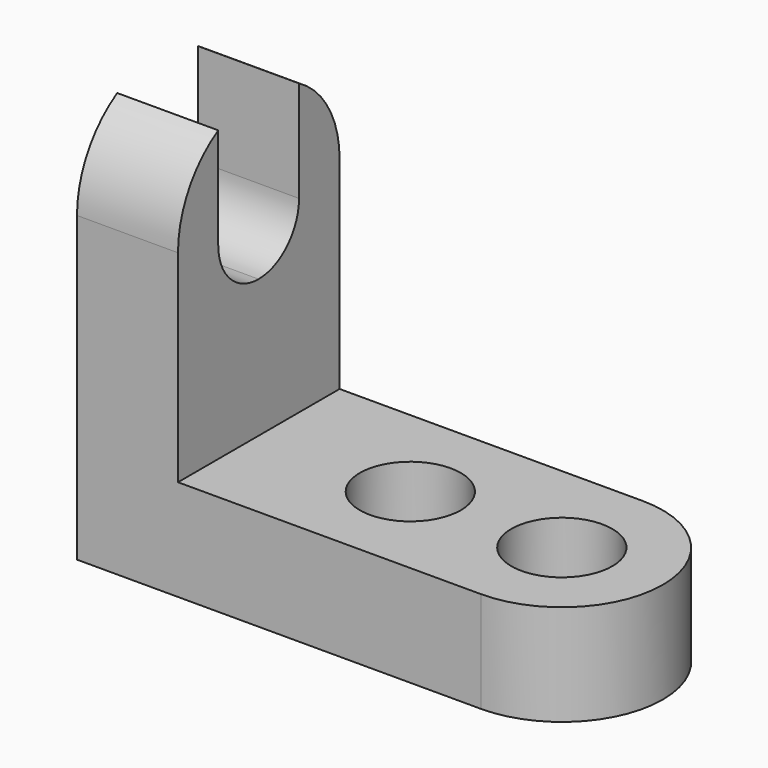
from build123d import *

# Parameters (mm, degrees)
F0_R        = 12.7
F1_DEPTH    = 25.4
F2_W        = 25.4
F2_H        = 50.8
F3_DEPTH    = 76.2
F4_R        = 25.4
F5_T1_DEPTH = 152.4
F7_DEPTH    = 25.401
F8_R        = 12.7
F9_R        = 12.69999


# Not quite as in the source:
# - a fillet or chamfer that OpenCascade refuses, or shapes differently, is made with other operations: its cross-section is extruded or revolved along the edge and cut away or added
# - a fillet or chamfer is up to 0.001 mm smaller than in the source, because OpenCascade refuses the exact size


with BuildPart() as f1:
    # F0 (on Top) → F1 (new body)
    with BuildSketch(Plane.XY):
        with BuildLine():
            Line((57.198610294, 38.3368320964), (-44.401389706, 38.3368320964))
            Line((-44.401389706, 38.3368320964), (-44.401389706, -12.4631679036))
            Line((-44.401389706, -12.4631679036), (57.198610294, -12.4631679036))
            ThreePointArc((57.198610294, -12.4631679036), (82.598610294, 12.9368320964), (57.198610294, 38.3368320964))
        make_face()
        with Locations((19.098610294, 12.9368320964)):
            Circle(F0_R, mode=Mode.SUBTRACT)
        with Locations((57.198610294, 12.9368320964)):
            Circle(F0_R, mode=Mode.SUBTRACT)
    extrude(amount=F1_DEPTH)

    # F2 (on face) → F3 (join)
    with BuildSketch(Plane.XY.offset(25.4)):
        with Locations((-31.701389706, 12.9368320964)):
            Rectangle(F2_W, F2_H)
    extrude(amount=F3_DEPTH)

    # F4
    f4_edges = [f1.edges().sort_by_distance(p)[0] for p in [
        (-31.70139, -12.463168, 101.6),
    ]]
    fillet(f4_edges, radius=F4_R)

    # F5: fillet of radius 25.4 on 1 edges, made by hand

    # F5_s2 → F5_t1 (cut)
    with BuildSketch(Plane.YZ.offset(-107.901389706)):
        with BuildLine():
            ThreePointArc((12.9368320964, 101.6), (30.8973443386, 94.1605122421), (38.3368320964, 76.2))
            Line((38.3368320964, 76.2), (38.3368320964, 101.6))
            Line((38.3368320964, 101.6), (12.9368320964, 101.6))
        make_face()
    extrude(amount=F5_T1_DEPTH, mode=Mode.SUBTRACT)

    # F6 (on face) → F7 (cut, through all)
    with BuildSketch(Plane.YZ.offset(-19.001389706)):
        with BuildLine():
            ThreePointArc((12.9368320964, 101.6), (6.3316674028, 100.7261452204), (0.1809873343, 98.1647086118))
            Line((0.1809873343, 98.1647086118), (0.1809873343, 60.0647086118))
            Line((0.1809873343, 60.0647086118), (25.5809873343, 60.0647086118))
            Line((25.5809873343, 60.0647086118), (25.5809873343, 98.2291928659))
            ThreePointArc((25.5809873343, 98.2291928659), (19.4797099497, 100.742834991), (12.9368320964, 101.6))
        make_face()
    extrude(amount=-F7_DEPTH, mode=Mode.SUBTRACT)

    # F8
    f8_edges = [f1.edges().sort_by_distance(p)[0] for p in [
        (-31.70139, 0.180987, 60.064709),
    ]]
    fillet(f8_edges, radius=F8_R)

    # F9 (radius 12.7 in the source; OpenCascade refuses exactly that, so slightly less here)
    f9_edges = [f1.edges().sort_by_distance(p)[0] for p in [
        (-31.70139, 25.580987, 60.064709),
    ]]
    fillet(f9_edges, radius=F9_R)


solid = f1.part
